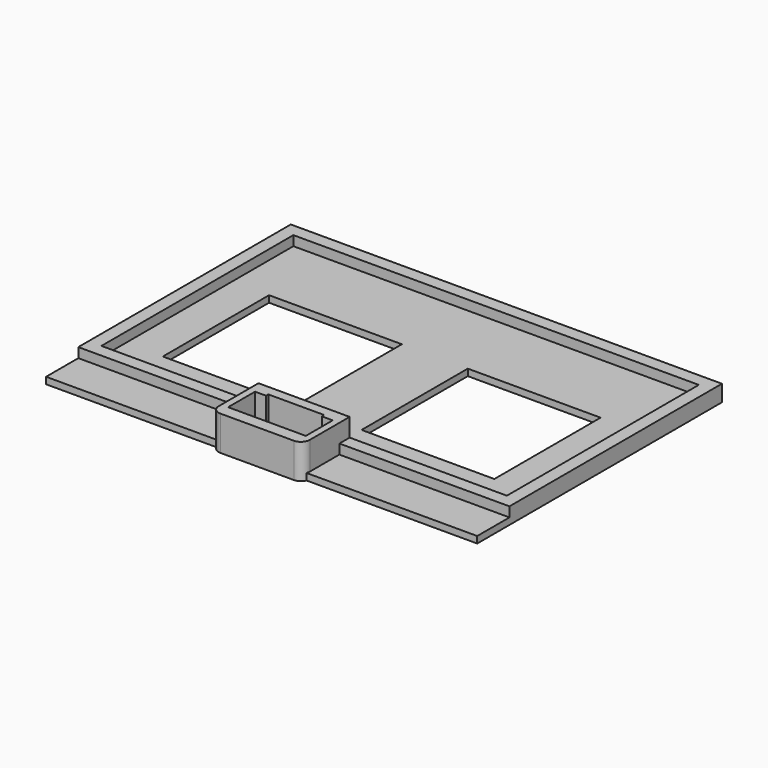
from build123d import *

# Parameters (mm, degrees)
F0_W     = 38.1
F0_H     = 38.1
F1_DEPTH = 1.905
F0_W_2   = 48.74895
F0_H_2   = 11.557
F0_W_3   = 48.79975
F2_DEPTH = 4.699
F0_W_4   = 13.589
F0_H_3   = 3.5052
F3_DEPTH = 9.9314
F4_R     = 2.54


# Not quite as in the source:
# - a feature names something its author has since deleted; it is built from what else it names


with BuildPart() as f1:
    # F0 (on Top) → F1 (new body)
    with BuildSketch(Plane.XY):
        Polygon((-13.10005, -34.417), (13.04925, -34.417), (58.166, -34.417), (58.166, 34.417), (-58.166, 34.417), (-58.166, -34.417), align=None)
        with Locations((-28.5115, -6.604)):
            Rectangle(F0_W, F0_H, mode=Mode.SUBTRACT)
        with Locations((28.5115, -6.604)):
            Rectangle(F0_W, F0_H, mode=Mode.SUBTRACT)
    extrude(amount=F1_DEPTH)



with BuildPart() as f1b:
    # F0 (on Top) → F1, piece 2 (new body)
    with BuildSketch(Plane.XY):
        with Locations((-37.474525, -43.8785)):
            Rectangle(F0_W_2, F0_H_2)
    extrude(amount=F1_DEPTH)


with BuildPart() as f1c:
    # F0 (on Top) → F1, piece 3 (new body)
    with BuildSketch(Plane.XY):
        with Locations((37.449125, -43.8785)):
            Rectangle(F0_W_3, F0_H_2)
    extrude(amount=F1_DEPTH)


with BuildPart() as f1_1:
    add(f1.part)

    add(f1b.part)  # F2 merges F1b

    add(f1c.part)  # F2 merges F1c
    # F0 (on Top) → F2 (join)
    with BuildSketch(Plane.XY):
        Polygon((61.849, -38.1), (61.849, 38.1), (-61.849, 38.1), (-61.849, -38.1), (-13.10005, -38.1), (-13.10005, -34.417), (-58.166, -34.417), (-58.166, 34.417), (58.166, 34.417), (58.166, -34.417), (13.04925, -34.417), (13.04925, -38.1), align=None)
    extrude(amount=F2_DEPTH)

    # F0 (on Top) → F3 (join)
    with BuildSketch(Plane.XY):
        Polygon((11.14425, -38.1), (13.04925, -38.1), (13.04925, -34.417), (-13.10005, -34.417), (-13.10005, -38.1), (-11.14425, -38.1), (-8.001, -38.1), (-8.001, -37.2745), (8.001, -37.2745), (8.001, -38.1), align=None)
        Polygon((-11.14425, -38.1), (-13.10005, -38.1), (-13.10005, -49.657), (-13.10005, -51.2572), (-6.7945, -51.2572), (-6.7945, -47.752), (-11.14425, -47.752), align=None)
        Polygon((13.04925, -49.657), (13.04925, -38.1), (11.14425, -38.1), (11.14425, -47.752), (6.7945, -47.752), (6.7945, -51.2572), (13.04925, -51.2572), align=None)
        with Locations((0, -49.5046)):
            Rectangle(F0_W_4, F0_H_3)
    extrude(amount=F3_DEPTH)

    # F4
    f4_edges = [f1_1.edges().sort_by_distance(p)[0] for p in [
        (-13.10005, -51.2572, 4.9657),
        (13.04925, -51.2572, 4.9657),
    ]]
    fillet(f4_edges, radius=F4_R)


solid = f1_1.part
